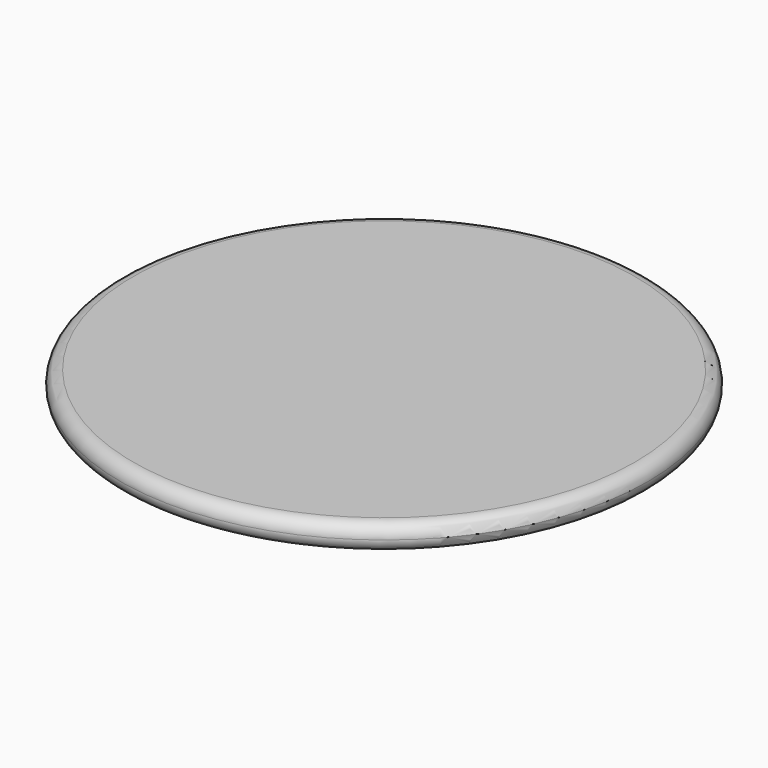
from build123d import *

# Parameters (mm, degrees)
F0_R     = 260
F1_DEPTH = 25.4
F2_R     = 12.69999
F3_R     = 4
F4_DEPTH = 19.05
F5_DEPTH = 19.05


# Not quite as in the source:
# - a fillet or chamfer is up to 0.001 mm smaller than in the source, because OpenCascade refuses the exact size


with BuildPart() as f1:
    # F0 (on Top) → F1 (new body)
    with BuildSketch(Plane.XY):
        Circle(F0_R)
    extrude(amount=F1_DEPTH)

    # F2 (radius 12.7 in the source; OpenCascade refuses exactly that, so slightly less here)
    f2_edges = [f1.edges().sort_by_distance(p)[0] for p in [
        (-260, 0, 25.4),
        (-260, 0, 0),
    ]]
    fillet(f2_edges, radius=F2_R)

    # F3 (on face) → F4 (cut)
    with BuildSketch(Plane(origin=(0, 0, 0), x_dir=(1, 0, 0), z_dir=(0, 0, -1))):
        with Locations((160.0338797814, 166.028664158)):
            Circle(F3_R)
    extrude(amount=-F4_DEPTH, mode=Mode.SUBTRACT)

    # F3 (on face) → F5 (cut)
    with BuildSketch(Plane(origin=(0, 0, 0), x_dir=(1, 0, 0), z_dir=(0, 0, -1))):
        with Locations((-160.0338797814, 166.028664158)):
            Circle(F3_R)
        with Locations((160.0338797814, 166.028664158)):
            Circle(F3_R)
        with Locations((160.0338797814, -166.028664158)):
            Circle(F3_R)
        with Locations((-160.0338797814, -166.028664158)):
            Circle(F3_R)
    extrude(amount=-F5_DEPTH, mode=Mode.SUBTRACT)


solid = f1.part
